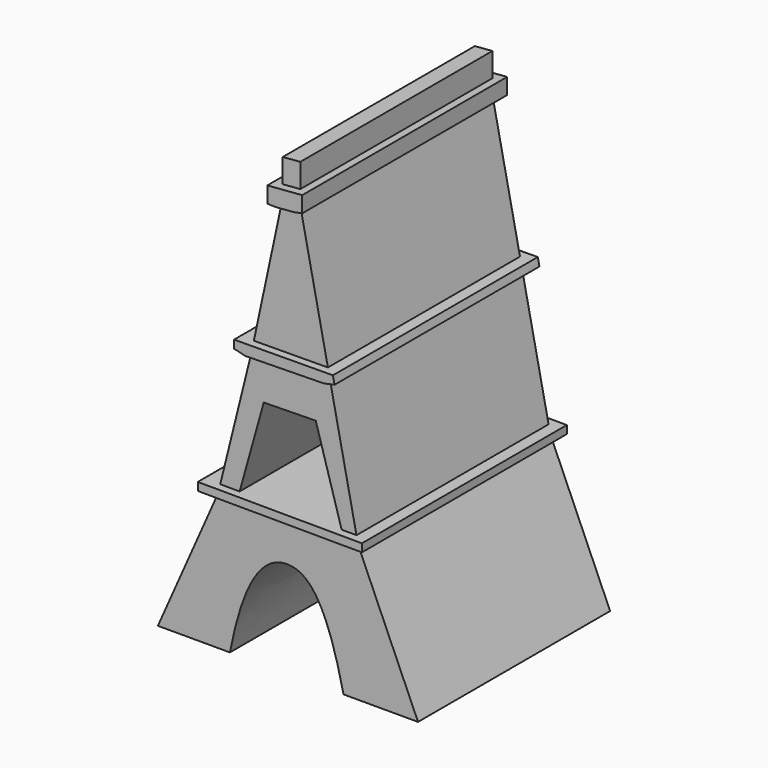
from build123d import *

# Parameters (mm, degrees)
F1_DEPTH = 3810
F2_DEPTH = 4064
F3_DEPTH = 4064


with BuildPart() as f1:
    # F0 (on Front) → F1 (new body, symmetric)
    with BuildSketch(Plane.XZ):
        Polygon((3962.2926947661, 14386.861276684), (3962.2926947661, 13624.861276684), (4519.3225083359, 13669.3048003329), (4519.3225083359, 14431.3048003329), align=None)
    extrude(amount=F1_DEPTH, both=True)


with BuildPart() as f1b:
    # F0 (on Front) → F1, piece 2 (new body, symmetric)
    with BuildSketch(Plane.XZ):
        Polygon((3927.887741484, 13082.1987645631), (3045.2767241419, 8955.0596301024), (5394.8737459492, 8971.7391000787), (4535.5270933105, 13131.0513807869), align=None)
    extrude(amount=F1_DEPTH, both=True)


with BuildPart() as f1c:
    # F0 (on Front) → F1, piece 3 (new body, symmetric)
    with BuildSketch(Plane.XZ):
        Polygon((2971.7602322705, 8611.2923479486), (1978.7751916019, 4599.6699502344), (2594.0482501344, 4597.0187600642), (3359.3227863312, 7331.6221237183), (5010.0841125311, 7359.6942437446), (5830.4841524302, 4583.0730705337), (6302.0264863643, 4581.0412110475), (5460.600385618, 8653.6164673729), align=None)
    extrude(amount=F1_DEPTH, both=True)

    # F0 (on Front) → F2 (join, symmetric)
    with BuildSketch(Plane.XZ):
        Polygon((1978.7751916019, 4599.6699502344), (1915.9703087599, 4345.9405742862), (6354.5516468159, 4326.8148819613), (6302.0264863643, 4581.0412110475), (5830.4841524302, 4583.0730705337), (2594.0482501344, 4597.0187600642), align=None)
        Polygon((1469.138337915, 4347.8659576788), (1915.9703087599, 4345.9405742862), (1978.7751916019, 4599.6699502344), (1469.138337915, 4601.8659576788), align=None)
        Polygon((6302.0264863643, 4581.0412110475), (6354.5516468159, 4326.8148819613), (6676.0899989331, 4325.4293844059), (6676.0899989331, 4579.4293844059), align=None)
    extrude(amount=F2_DEPTH, both=True)


with BuildPart() as f1d:
    # F0 (on Front) → F1, piece 4 (new body, symmetric)
    with BuildSketch(Plane.XZ):
        with BuildLine():
            Line((1909.8379015153, 4321.1658785489), (0, 0))
            Line((0, 0), (2286, 0))
            add(Edge.make_bspline(
                [(2286, 0), (2759.3298407348, 2457.1255667936), (4156.1876931975, 3664.5077452441), (5350.7589243341, 2441.5044118267), (5892.8, 0)],
                knots=[0, 0, 0, 0, 0.5006396986, 1, 1, 1, 1], degree=3))
            Line((5892.8, 0), (8255, 0))
            Line((8255, 0), (6354.8379015153, 4325.4293844059))
            Line((6354.8379015153, 4325.4293844059), (1909.8379015153, 4321.1658785489))
        make_face()
    extrude(amount=F1_DEPTH, both=True)


with BuildPart() as f3:
    # F0 (on Front) → F3 (new body, symmetric)
    with BuildSketch(Plane.XZ):
        Polygon((3045.2767241419, 8955.0596301024), (2971.7602322705, 8611.2923479486), (5460.600385618, 8653.6164673729), (5394.8737459492, 8971.7391000787), align=None)
        Polygon((5394.8737459492, 8971.7391000787), (5460.600385618, 8653.6164673729), (5808.845323328, 8725.5666123301), (5757.4523626443, 8974.3129964087), align=None)
        Polygon((2621.2640921677, 8698.0496220461), (2971.7602322705, 8611.2923479486), (3045.2767241419, 8955.0596301024), (2621.2640921677, 8952.0496220461), align=None)
    extrude(amount=F3_DEPTH, both=True)


with BuildPart() as f3b:
    # F0 (on Front) → F3, piece 2 (new body, symmetric)
    with BuildSketch(Plane.XZ):
        Polygon((3674.1561126888, 13093.8718339509), (3927.887741484, 13082.1987645631), (4535.5270933105, 13131.0513807869), (4784.2734773891, 13182.4443414707), (4784.2734773891, 13690.4443414707), (4519.3225083359, 13669.3048003329), (3962.2926947661, 13624.861276684), (3674.1561126888, 13601.8718339509), align=None)
    extrude(amount=F3_DEPTH, both=True)


solid = Compound([f1.part, f1b.part, f1c.part, f1d.part, f3.part, f3b.part])
